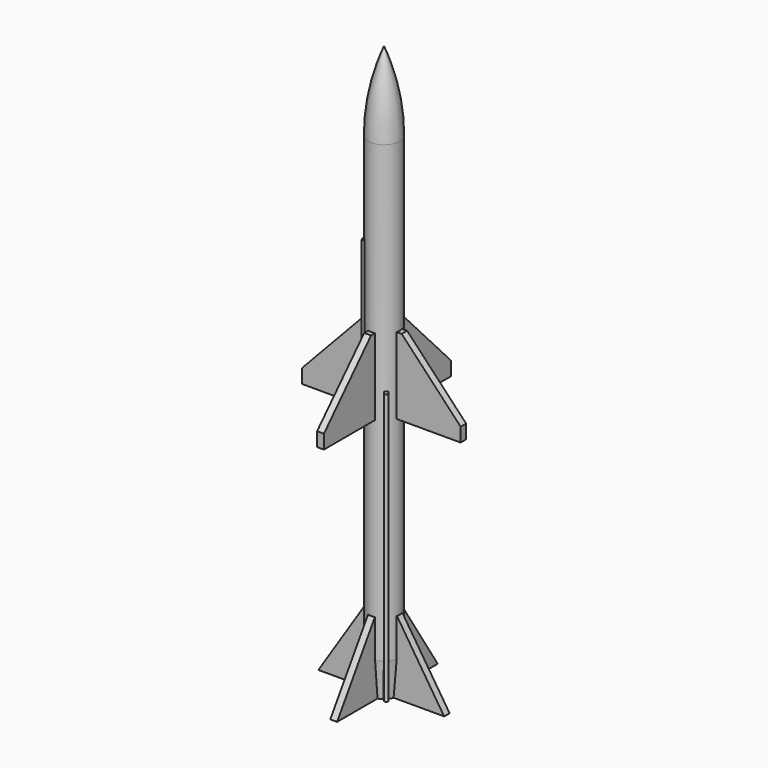
from build123d import *

# Parameters (mm, degrees)
F5_DEPTH      = 0.1524
F6_COUNT      = 4
F8_DEPTH      = 3.3506944444
F10_DEPTH     = 12.0833333333
F11_T4_ANGLE  = 55.3885988596
F11_S5_R      = 0.0834798304
F11_T6_DEPTH  = 2
F11_T10_ANGLE = 55.3885988596
F11_S11_R     = 0.0834798304
F11_T12_DEPTH = 2
F11_T16_ANGLE = 55.3885988596
F11_S17_R     = 0.0833333333
F11_T18_DEPTH = 2


# Not quite as in the source:
# - a fillet or chamfer that OpenCascade refuses, or shapes differently, is made with other operations: its cross-section is extruded or revolved along the edge and cut away or added


with BuildPart() as f1:
    # F0 (on Front) → F1 (revolve)
    with BuildSketch(Plane.XZ):
        with BuildLine():
            Line((0, 25.4166666667), (0, 0))
            Line((0, 0), (0.7048611111, 0))
            Line((0.7048611111, 0), (0.7048611111, 21.8958333333))
            ThreePointArc((0.7048611111, 21.8958333333), (0.5269147233, 23.6911812486), (0, 25.4166666667))
        make_face()
    revolve(axis=Axis((0, 0, 12.7083333333), (0, 0, 1)))

    # F2 (on Front) → F3 (revolve, cut)
    with BuildSketch(Plane.XZ):
        Polygon((0.7048611111, 1.5625), (0.5729166667, 0), (0.7048611111, 0), (1.5729166667, 0), (1.5729166667, 1.5625), align=None)
    revolve(axis=Axis((0, 0, 0), (0, 0, 1)), mode=Mode.SUBTRACT)

    # F4 (on Front) → F5 (join, symmetric)
    with BuildSketch(Plane.XZ):
        Polygon((0.7048611111, 14.4444444444), (-0.7048611111, 14.4444444444), (-0.9131944444, 14.4444444444), (-3.5498263889, 11.6464416667), (-3.5498263889, 11.0214416667), (-0.7048611111, 11.0214416667), (0.7048611111, 11.0214416667), (3.5498263889, 11.0214416667), (3.5498263889, 11.6464416667), (0.9131944444, 14.4444444444), align=None)
        Polygon((2.8125, 0), (0.7048611111, 3.2631944444), (-0.7048611111, 3.2631944444), (-2.8125, 0), (-0.1651, 0), (0.1651, 0), align=None)
    extrude(amount=F5_DEPTH, both=True)

    # F6: F1 ×4 about axis
    f6_axis = Axis((0, 0, 0), (0, 0, 1))


with BuildPart() as f1_1:
    add(f1.part)
    for i in range(1, F6_COUNT):
        add(f1.part.rotate(f6_axis, i * 360 / F6_COUNT))

    # F7 (on face) → F8 (join, symmetric)
    with BuildSketch(Plane.XY.offset(14.4444444444)):
        with BuildLine():
            ThreePointArc((-0.5538420942, -0.435990964), (-0.5574412256, -0.5574412256), (-0.435990964, -0.5538420942))
            ThreePointArc((-0.435990964, -0.5538420942), (-0.4984120715, -0.4984120715), (-0.5538420942, -0.435990964))
        make_face()
        with BuildLine():
            ThreePointArc((-0.5538420942, -0.435990964), (-0.4984120715, -0.4984120715), (-0.435990964, -0.5538420942))
            Line((-0.435990964, -0.5538420942), (-0.3224915619, -0.4403426921))
            Line((-0.3224915619, -0.4403426921), (-0.4403426921, -0.3224915619))
            Line((-0.4403426921, -0.3224915619), (-0.5538420942, -0.435990964))
        make_face()
    extrude(amount=F8_DEPTH, both=True)

    # F9 (on face) → F10 (join)
    with BuildSketch(Plane(origin=(0, 0, 0), x_dir=(1, 0, 0), z_dir=(0, 0, -1))):
        with BuildLine():
            ThreePointArc((0.435990964, 0.5538420942), (0.4984120715, 0.4984120715), (0.5538420942, 0.435990964))
            ThreePointArc((0.5538420942, 0.435990964), (0.5538420942, 0.5538420942), (0.435990964, 0.5538420942))
        make_face()
        with BuildLine():
            ThreePointArc((0.3418792892, 0.4597304194), (0.4051132601, 0.4051132601), (0.4597304194, 0.3418792892))
            Line((0.4597304194, 0.3418792892), (0.5538420942, 0.435990964))
            ThreePointArc((0.5538420942, 0.435990964), (0.4984120715, 0.4984120715), (0.435990964, 0.5538420942))
            Line((0.435990964, 0.5538420942), (0.3418792892, 0.4597304194))
        make_face()
    extrude(amount=-F10_DEPTH)

    # F11: chamfer of 0.1 on 3 edges, made by hand


with BuildPart() as f11_tool2:
    # F11_s3 → F11_t4 (revolve)
    with BuildSketch(Plane(origin=(0, 0, 0), x_dir=(0, 0, 1), z_dir=(-0.2974698653, 0.9547312078, 0))):
        Polygon((17.8951388889, -0.7048611111), (17.7951388889, -0.8048611111), (17.7951388889, -0.7048611111), align=None)
    revolve(axis=Axis((0, 0, 17.7951388889), (0, 0, 1)), revolution_arc=F11_T4_ANGLE)

    # F11_s5 → F11_t6 (intersect, symmetric)
    with BuildSketch(Plane.XY.offset(17.8)):
        with Locations((-0.4984120715, -0.4984120715)):
            Circle(F11_S5_R)
    extrude(amount=F11_T6_DEPTH, both=True, mode=Mode.INTERSECT)


with BuildPart() as f1_2:
    add(f1_1.part)

    # F11_t1: union F11_tool2
    add(f11_tool2.part)


with BuildPart() as f11_tool8:
    # F11_s9 → F11_t10 (revolve)
    with BuildSketch(Plane(origin=(0, 0, 0), x_dir=(0, 0, 1), z_dir=(-0.2974698653, 0.9547312078, 0))):
        Polygon((10.99375, -0.7048611111), (11.09375, -0.8048611111), (11.09375, -0.7048611111), align=None)
    revolve(axis=Axis((0, 0, 11.09375), (0, 0, 1)), revolution_arc=F11_T10_ANGLE)

    # F11_s11 → F11_t12 (intersect, symmetric)
    with BuildSketch(Plane.XY.offset(11)):
        with Locations((-0.4984120715, -0.4984120715)):
            Circle(F11_S11_R)
    extrude(amount=F11_T12_DEPTH, both=True, mode=Mode.INTERSECT)


with BuildPart() as f1_3:
    add(f1_2.part)

    # F11_t7: union F11_tool8
    add(f11_tool8.part)


with BuildPart() as f11_tool14:
    # F11_s15 → F11_t16 (revolve)
    with BuildSketch(Plane(origin=(0, 0, 0), x_dir=(0, 0, 1), z_dir=(-0.9547312078, -0.2974698653, 0))):
        Polygon((12.1833333333, -0.7048611111), (12.0833333333, -0.8048611111), (12.0833333333, -0.7048611111), align=None)
    revolve(axis=Axis((0, 0, 12.0833333333), (0, 0, 1)), revolution_arc=F11_T16_ANGLE)

    # F11_s17 → F11_t18 (intersect, symmetric)
    with BuildSketch(Plane.XY.offset(12.1)):
        with Locations((0.4949165291, -0.4949165291)):
            Circle(F11_S17_R)
    extrude(amount=F11_T18_DEPTH, both=True, mode=Mode.INTERSECT)


with BuildPart() as f1_4:
    add(f1_3.part)

    # F11_t13: union F11_tool14
    add(f11_tool14.part)


solid = f1_4.part
